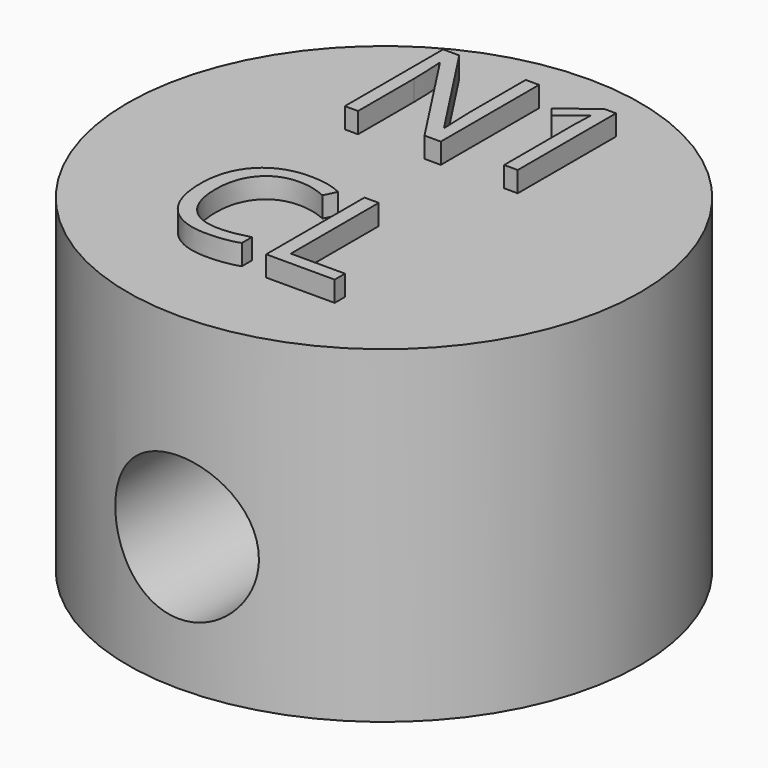
from build123d import *

# Parameters (mm, degrees)
F0_R         = 12.5
F1_DEPTH     = 16
F3_R         = 3.5
F4_DEPTH     = 25.001
F5_TEXT_SIZE = 8.3901415836
F6_DEPTH     = 1


# Not quite as in the source:
# - Text() gives the source's letters only with a copy of the font that has no kerning and outlines rounded to 1/6400 em; it was checked with that copy


with BuildPart() as f1:
    # F0 (on Top) → F1 (new body)
    with BuildSketch(Plane.XY):
        Circle(F0_R)
    extrude(amount=F1_DEPTH)

    # F3 (on offset) → F4 (cut, through all)
    with BuildSketch(Plane.XZ.offset(-12.5)):
        with Locations((0, 6.5)):
            Circle(F3_R)
    extrude(amount=F4_DEPTH, mode=Mode.SUBTRACT)

    # F5 (on face) → F6 (join)
    with BuildSketch(Plane.XY.offset(16)):
        with Locations((-5.5, 3.4590980598)):
            Text('N1', F5_TEXT_SIZE, font='Open Sans', text_align=(TextAlign.LEFT, TextAlign.BOTTOM))
        with Locations((-5.5, -7.951494494)):
            Text('CL', F5_TEXT_SIZE, font='Open Sans', text_align=(TextAlign.LEFT, TextAlign.BOTTOM))
    extrude(amount=F6_DEPTH)


solid = f1.part
